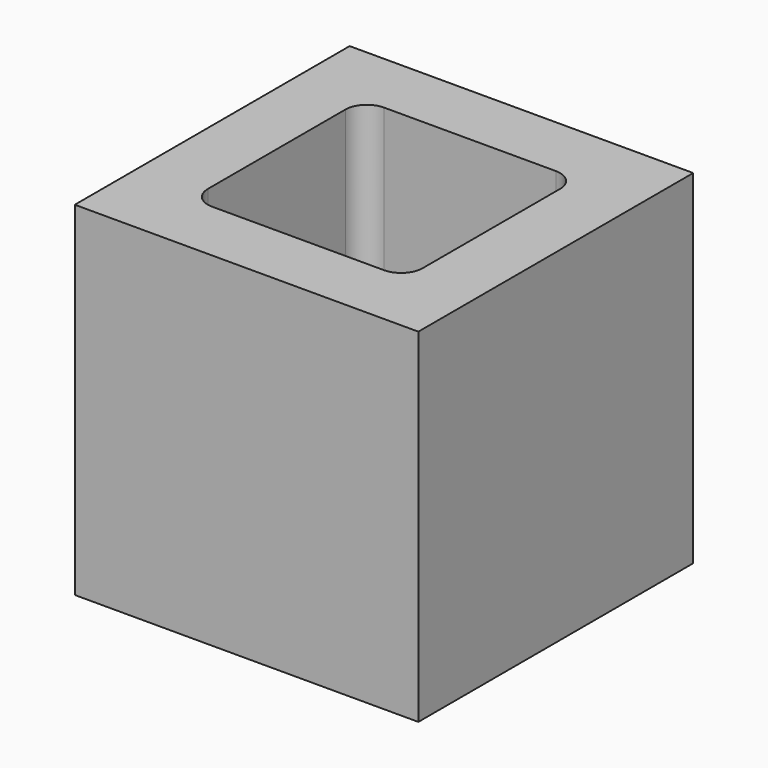
from build123d import *

# Parameters (mm, degrees)
F1_W     = 203.2
F1_H     = 203.2
F2_DEPTH = 203.2


# Not quite as in the source:
# - a variable given as a bare number and used for a length is read in inches; the dataset says mm whatever the document's units were


with BuildPart() as f2:
    # F1 (on Top) → F2 (new body)
    with BuildSketch(Plane.XY):
        Rectangle(F1_W, F1_H)
        with BuildLine():
            Line((-50.8, 63.5), (50.8, 63.5))
            ThreePointArc((50.8, 63.5), (59.7802561211, 59.7802561211), (63.5, 50.8))
            Line((63.5, 50.8), (63.5, -50.8))
            ThreePointArc((63.5, -50.8), (59.7802561211, -59.7802561211), (50.8, -63.5))
            Line((50.8, -63.5), (-50.8, -63.5))
            ThreePointArc((-50.8, -63.5), (-59.7802561211, -59.7802561211), (-63.5, -50.8))
            Line((-63.5, -50.8), (-63.5, 50.8))
            ThreePointArc((-63.5, 50.8), (-59.7802561211, 59.7802561211), (-50.8, 63.5))
        make_face(mode=Mode.SUBTRACT)
    extrude(amount=F2_DEPTH)


solid = f2.part
